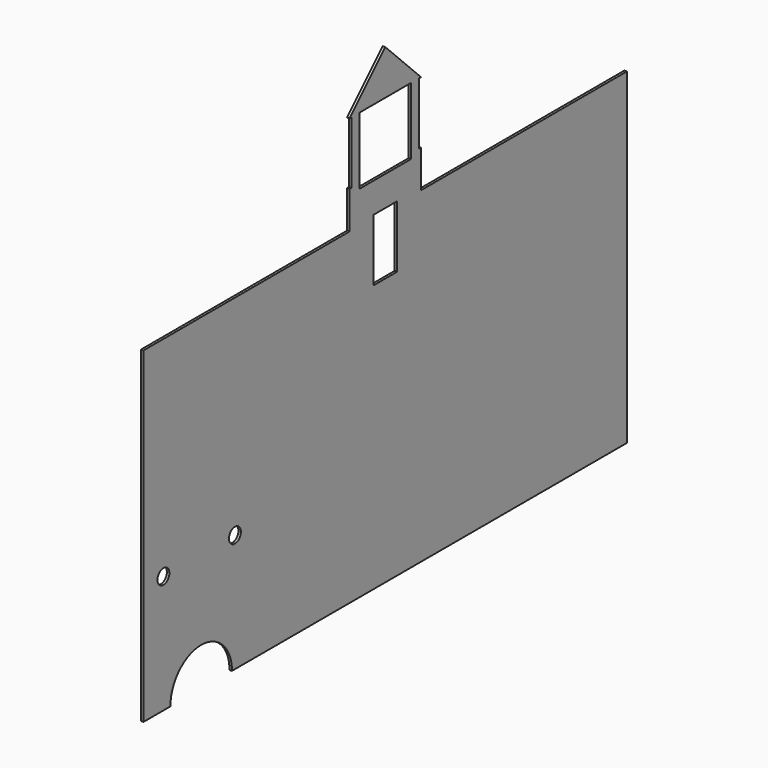
from build123d import *

# Parameters (mm, degrees)
F0_W     = 19.65
F0_H     = 1.5
F1_DEPTH = 1


# Not quite as in the source:
# - a feature names something its author has since deleted; it is built from what else it names


with BuildPart() as f1:
    # F0 (on Right) → F1 (new body)
    with BuildSketch(Plane.YZ):
        Polygon((121.65, -16.375), (19.65, -16.375), (-19.65, -16.375), (-61.65, -16.375), (-61.65, -39.125), (121.65, -39.125), align=None)
        Polygon((-19.65, -16.375), (19.65, -16.375), (19.65, 14.875), (0, 14.875), (-19.65, 14.875), align=None)
        Polygon((19.65, 14.875), (19.65, -16.375), (121.65, -16.375), (121.65, 16.375), (19.65, 16.375), align=None)
        Polygon((-61.65, -16.375), (-19.65, -16.375), (-19.65, 14.875), (-19.65, 16.375), (-19.65, 57.475), (-19.65, 92.575), (-121.65, 92.575), (-121.65, 89.375), (-121.65, 16.375), (-111.65, 16.375), (-75.65, 16.375), (-61.65, 16.375), align=None)
        with Locations((9.825, 15.625)):
            Rectangle(F0_W, F0_H)
        with Locations((-9.825, 15.625)):
            Rectangle(F0_W, F0_H)
        with BuildLine():
            Line((-61.65, -39.125), (-61.65, -16.375))
            Line((-61.65, -16.375), (-121.65, -16.375))
            Line((-121.65, -16.375), (-121.65, -39.125))
            Line((-121.65, -39.125), (-111.65, -39.125))
            ThreePointArc((-111.65, -39.125), (-92.65, -20.125), (-73.65, -39.125))
            Line((-73.65, -39.125), (-61.65, -39.125))
        make_face()
        Polygon((-121.65, -16.375), (-61.65, -16.375), (-61.65, 16.375), (-75.65, 16.375), (-111.65, 16.375), (-121.65, 16.375), align=None)
        with BuildLine():
            ThreePointArc((-108.65, 8.375), (-113.7713203436, 6.2536796564), (-111.65, 11.375))
            ThreePointArc((-111.65, 11.375), (-109.5286796564, 10.4963203436), (-108.65, 8.375))
        make_face(mode=Mode.SUBTRACT)
        with BuildLine():
            ThreePointArc((-72.65, 8.375), (-77.7713203436, 6.2536796564), (-75.65, 11.375))
            ThreePointArc((-75.65, 11.375), (-73.5286796564, 10.4963203436), (-72.65, 8.375))
        make_face(mode=Mode.SUBTRACT)
        Polygon((19.65, 57.475), (19.65, 16.375), (121.65, 16.375), (121.65, 89.375), (121.65, 92.575), (19.65, 92.575), align=None)
        Polygon((0, 16.375), (19.65, 16.375), (19.65, 57.475), (6, 57.475), (6, 29.475), (0, 29.475), align=None)
        Polygon((-19.65, 57.475), (-19.65, 16.375), (0, 16.375), (0, 29.475), (-6, 29.475), (-6, 57.475), align=None)
        Polygon((6, 57.475), (19.65, 57.475), (19.65, 92.575), (18, 92.575), (18, 105.675), (18, 107.675), (17, 107.675), (17, 132.675), (18, 132.675), (0, 150.675), (0, 132.675), (13, 132.675), (13, 105.675), (0, 105.675), (0, 93.575), (6, 93.575), (6, 92.575), (6, 89.375), (6, 70.575), (6, 68.575), align=None)
        Polygon((-19.65, 92.575), (-19.65, 57.475), (-6, 57.475), (-6, 29.475), (0, 29.475), (6, 29.475), (6, 57.475), (6, 68.575), (-6, 68.575), (-6, 70.575), (-6, 92.575), (-6, 93.575), (0, 93.575), (0, 105.675), (-13, 105.675), (-13, 132.675), (0, 132.675), (0, 150.675), (-18, 132.675), (-17, 132.675), (-17, 107.675), (-18, 107.675), (-18, 105.675), (-18, 92.575), align=None)
        with BuildLine():
            Line((-77.15, -39.125), (-73.65, -39.125))
            ThreePointArc((-73.65, -39.125), (-92.65, -20.125), (-111.65, -39.125))
            Line((-111.65, -39.125), (-108.15, -39.125))
            ThreePointArc((-108.15, -39.125), (-92.65, -23.625), (-77.15, -39.125))
        make_face()
    extrude(amount=F1_DEPTH)


solid = f1.part
